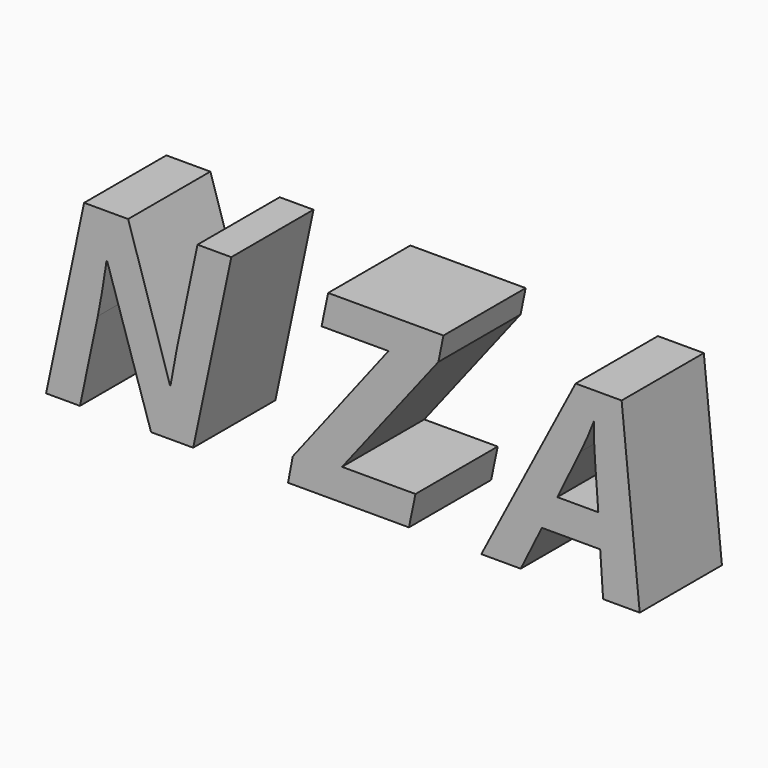
from build123d import *

# Parameters (mm, degrees)
F0_TEXT_SIZE = 24.5571401164
F1_DEPTH     = 10


# Not quite as in the source:
# - Text() gives the source's letters only with a copy of the font that has no kerning and outlines rounded to 1/6400 em; it was checked with that copy


with BuildPart() as f1:
    # F0 (on Front) → F1 (new body)
    with BuildSketch(Plane.XZ):
        with Locations((-6.4645875649, 1.5211191876)):
            Text('N Z A', F0_TEXT_SIZE, font='Open Sans', font_style=FontStyle.BOLDITALIC, text_align=(TextAlign.LEFT, TextAlign.BOTTOM))
    extrude(amount=F1_DEPTH)


solid = f1.part
